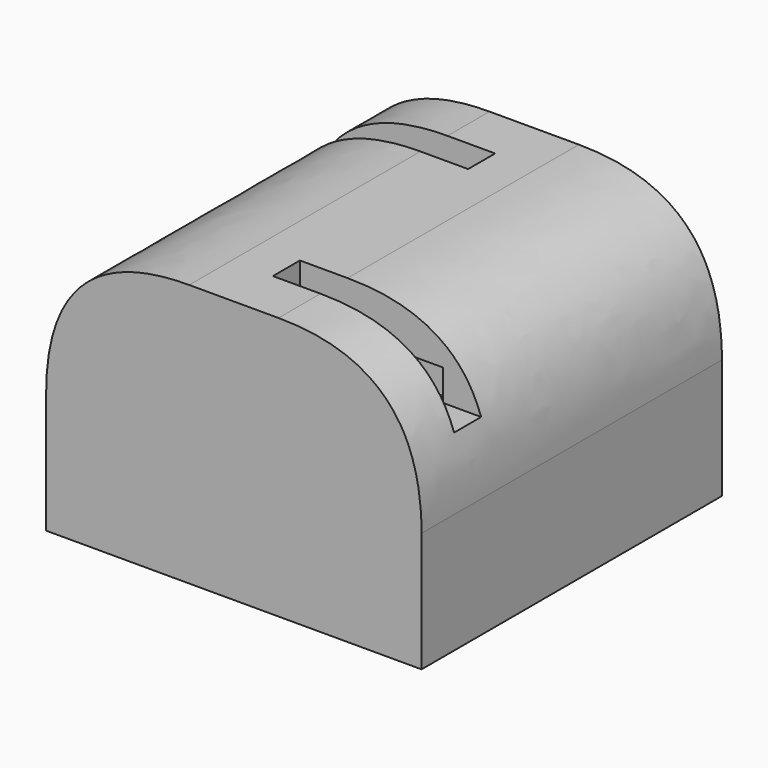
from build123d import *

# Parameters (mm, degrees)
F0_W        = 100
F0_H        = 70
F1_DEPTH    = 100
F2_T        = -12.7
F3_T1_DEPTH = 290.5
F4_T1_DEPTH = 290.5
F5_W        = 9
F5_H        = 32
F6_DEPTH    = 50.8
F7_W        = 9
F7_H        = 30
F8_DEPTH    = 50.8
F9_W        = 10
F9_H        = 10
F12_DEPTH   = 83.82


# Not quite as in the source:
# - a fillet or chamfer that OpenCascade refuses, or shapes differently, is made with other operations: its cross-section is extruded or revolved along the edge and cut away or added
# - a feature of the source that left no trace in its solid (it failed there, or was rolled back) is left out


with BuildPart() as f1:
    # F0 (on Front) → F1 (new body)
    with BuildSketch(Plane.XZ):
        with Locations((-15.9141167998, -52.9208671927)):
            Rectangle(F0_W, F0_H)
    extrude(amount=F1_DEPTH)

    # F2
    f2_openings = [f1.faces().sort_by_distance(p)[0] for p in [
        (-15.914117, -50, -87.920867),
    ]]
    offset(amount=F2_T, openings=f2_openings)

    # F3: fillet of radius 38.1 on 1 edges, made by hand

    # F3_s2 → F3_t1 (cut)
    with BuildSketch(Plane.XZ.offset(-95.25)):
        with BuildLine():
            add(Edge.make_bspline(
                [(34.0858832002, -56.0208671927), (34.0858832002, -17.9208671927), (-4.0141167998, -17.9208671927)],
                knots=[0, 0, 0, 1, 1, 1], degree=2, weights=[1, 1, 1]))
            Line((-4.0141167998, -17.9208671927), (34.0858832002, -17.9208671927))
            Line((34.0858832002, -17.9208671927), (34.0858832002, -56.0208671927))
        make_face()
    extrude(amount=F3_T1_DEPTH, mode=Mode.SUBTRACT)

    # F4: fillet of radius 38.1 on 1 edges, made by hand

    # F4_s2 → F4_t1 (cut)
    with BuildSketch(Plane.XZ.offset(-95.25)):
        with BuildLine():
            add(Edge.make_bspline(
                [(-27.8141167998, -17.9208671927), (-65.9141167998, -17.9208671927), (-65.9141167998, -56.0208671927)],
                knots=[0, 0, 0, 1, 1, 1], degree=2, weights=[1, 1, 1]))
            Line((-65.9141167998, -56.0208671927), (-65.9141167998, -17.9208671927))
            Line((-65.9141167998, -17.9208671927), (-27.8141167998, -17.9208671927))
        make_face()
    extrude(amount=F4_T1_DEPTH, mode=Mode.SUBTRACT)

    # F5 (on face) → F6 (cut)
    with BuildSketch(Plane(origin=(-65.9141167998, 0, 0), x_dir=(0, -1, 0), z_dir=(-1, 0, 0))):
        with Locations((18.5, -22.9208671927)):
            Rectangle(F5_W, F5_H)
    extrude(amount=-F6_DEPTH, mode=Mode.SUBTRACT)

    # F7 (on face) → F8 (cut)
    with BuildSketch(Plane.YZ.offset(34.0858832002)):
        with Locations((-81.5, -23.9208671927)):
            Rectangle(F7_W, F7_H)
    extrude(amount=-F8_DEPTH, mode=Mode.SUBTRACT)

    # F9 (on face) → F12 (join)
    with BuildSketch(Plane(origin=(21.3858832002, 0, 0), x_dir=(0, -1, 0), z_dir=(-1, 0, 0))):
        with Locations((25, -46.9208671927)):
            Rectangle(F9_W, F9_H)
        with Locations((75, -46.9208671927)):
            Rectangle(F9_W, F9_H)
    extrude(amount=F12_DEPTH)


solid = f1.part
